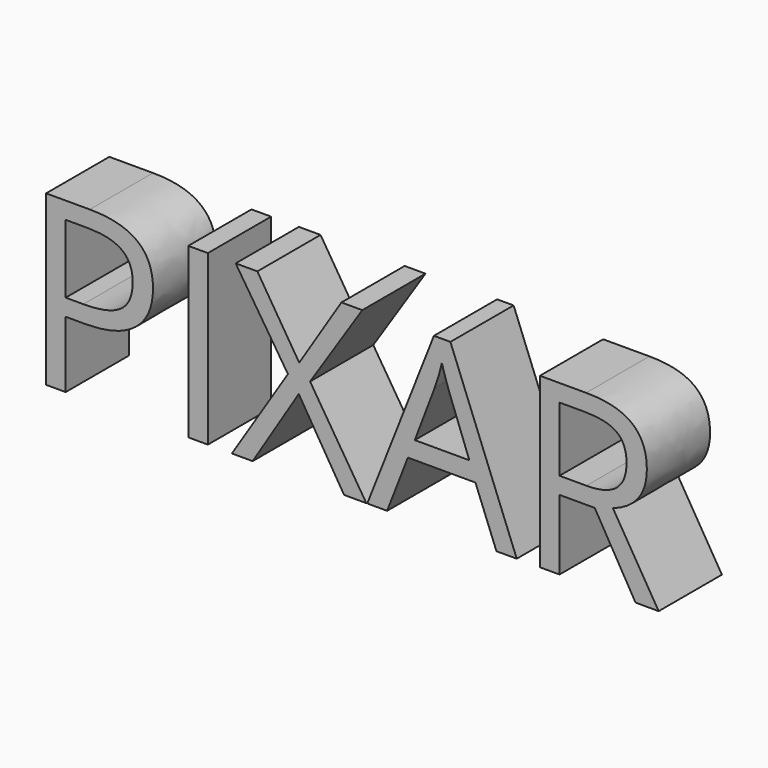
from build123d import *

# Parameters (mm, degrees)
F0_TEXT_SIZE = 144.2537022134
F1_DEPTH     = 48.26


# Not quite as in the source:
# - Text() gives the source's letters only with a copy of the font that has no kerning and outlines rounded to 1/6400 em; it was checked with that copy


with BuildPart() as f1:
    # F0 (on Front) → F1 (new body)
    with BuildSketch(Plane.XZ):
        with Locations((-66.5138810873, -36.2683087587)):
            Text('PIXAR', F0_TEXT_SIZE, font='Open Sans', text_align=(TextAlign.LEFT, TextAlign.BOTTOM))
    extrude(amount=F1_DEPTH)


solid = f1.part
